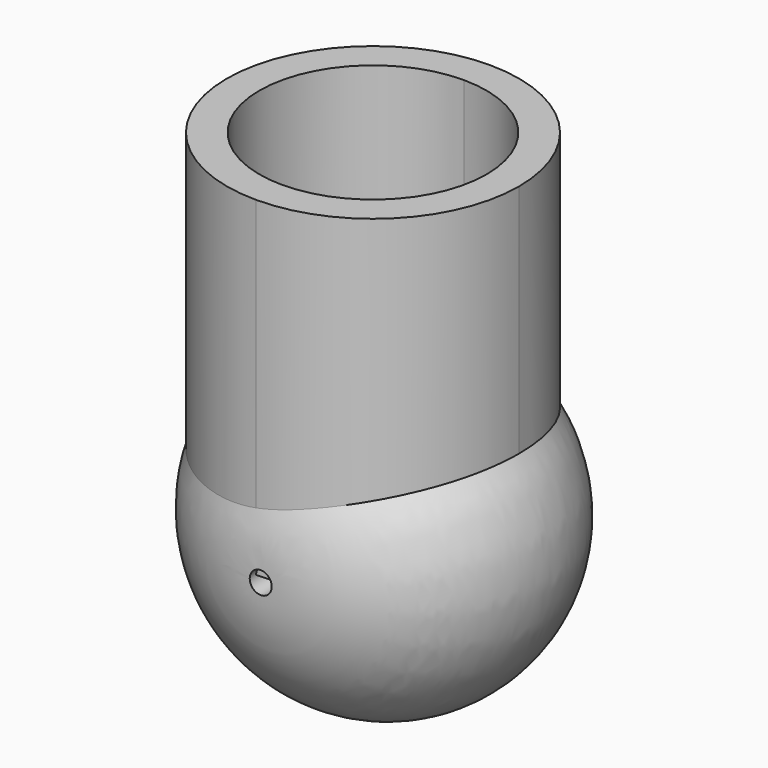
from build123d import *

# Parameters (mm, degrees)
F2_D     = 24.60625
F2_DEPTH = 90
F2_TIP   = 7.3924633035
F3_DEPTH = 30


# Not quite as in the source:
# - a length typed as a fraction of an inch, garbled in the dataset ("3 / 203.2 mm" for 3/8 in), is restored


with BuildPart() as f1:
    # F0 (on Top) → F1 (revolve)
    with BuildSketch(Plane.XY):
        with BuildLine():
            ThreePointArc((82.6243460178, -33.9253438014), (68.6243460178, -47.9253438014), (82.6243460178, -61.9253438014))
            Line((82.6243460178, -61.9253438014), (82.6243460178, -61.1992254835))
            ThreePointArc((82.6243460178, -61.1992254835), (69.3504643358, -47.9253438014), (82.6243460178, -34.6514621193))
            Line((82.6243460178, -34.6514621193), (82.6243460178, -33.9253438014))
        make_face()
        with BuildLine():
            ThreePointArc((82.6243460178, -34.6514621193), (69.3504643358, -47.9253438014), (82.6243460178, -61.1992254835))
            Line((82.6243460178, -61.1992254835), (82.6243460178, -58.2440938014))
            ThreePointArc((82.6243460178, -58.2440938014), (72.3055960178, -47.9253438014), (82.6243460178, -37.6065938014))
            Line((82.6243460178, -37.6065938014), (82.6243460178, -34.6514621193))
        make_face()
    revolve(axis=Axis((83.6243460178, -0.4812479019, 0), (0, 1, 0)))

    # F2 (one way)
    with BuildSketch(Plane(origin=(0, 0, 0), x_dir=(1, 0, 0), z_dir=(0, 0, -1))):
        with Locations((82.6243460178, 47.9253438014)):
            Circle(F2_D / 2)
    extrude(amount=-F2_DEPTH, mode=Mode.SUBTRACT)
    with Locations(Plane(origin=(0, 0, 0), x_dir=(1, 0, 0), z_dir=(0, 0, -1))):
        with Locations((82.6243460178, 47.9253438014)):
            with Locations((0, 0, -(F2_DEPTH + F2_TIP / 2))):  # 118° drill point
                Cone(0, F2_D / 2, F2_TIP, mode=Mode.SUBTRACT)

    # F0 (on Top) → F3 (join)
    with BuildSketch(Plane.XY):
        with BuildLine():
            ThreePointArc((82.6243460178, -34.6514621193), (69.3504643358, -47.9253438014), (82.6243460178, -61.1992254835))
            Line((82.6243460178, -61.1992254835), (82.6243460178, -58.2440938014))
            ThreePointArc((82.6243460178, -58.2440938014), (72.3055960178, -47.9253438014), (82.6243460178, -37.6065938014))
            Line((82.6243460178, -37.6065938014), (82.6243460178, -34.6514621193))
        make_face()
        with BuildLine():
            Line((82.6243460178, -58.2440938014), (82.6243460178, -61.1992254835))
            ThreePointArc((82.6243460178, -61.1992254835), (92.0103977679, -57.3113955515), (95.8982276999, -47.9253438014))
            ThreePointArc((95.8982276999, -47.9253438014), (92.0103977679, -38.5392920513), (82.6243460178, -34.6514621193))
            Line((82.6243460178, -34.6514621193), (82.6243460178, -37.6065938014))
            ThreePointArc((82.6243460178, -37.6065938014), (89.9208041162, -40.628885703), (92.9430960178, -47.9253438014))
            ThreePointArc((92.9430960178, -47.9253438014), (89.9208041162, -55.2218018998), (82.6243460178, -58.2440938014))
        make_face()
    extrude(amount=F3_DEPTH)


solid = f1.part
